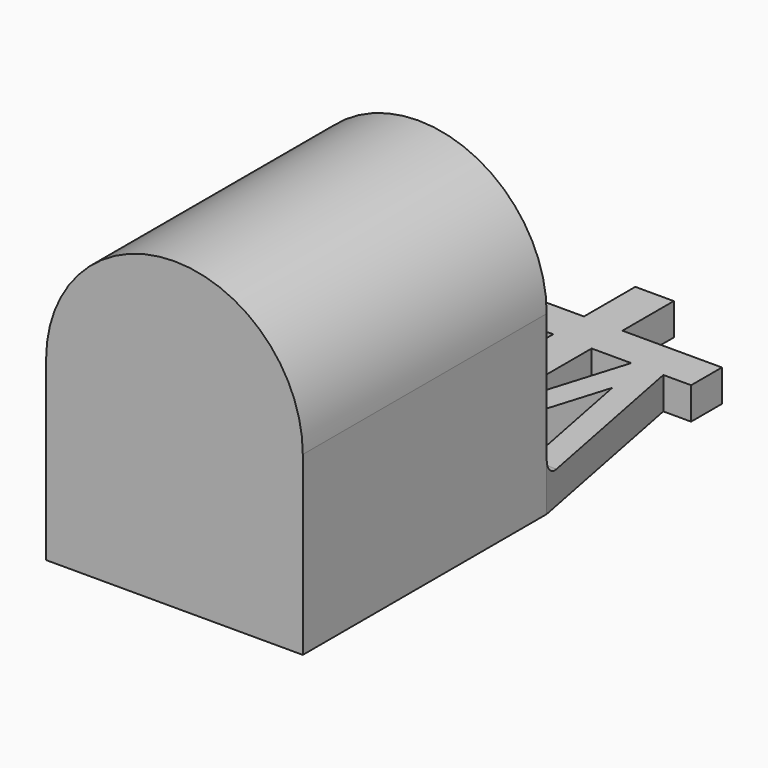
from build123d import *

# Parameters (mm, degrees)
F1_DEPTH  = 10
F3_DEPTH  = 100
F4_R      = 35
F5_DEPTH  = 90
F6_DEPTH  = 95.001
F7_R      = 5
F10_R     = 4
F11_DEPTH = 18


with BuildPart() as f1:
    # F0 (on Top) → F1 (new body)
    with BuildSketch(Plane.XY):
        Polygon((-6, 61.6815258077), (-6, 41.6815258077), (-37, 41.6815258077), (-37, 29.6815258077), (-28.3371814517, 29.6815258077), (-40, -30.3184741923), (-40, -125.3184741923), (0, -125.3184741923), (40, -125.3184741923), (40, -30.3184741923), (28.3371814517, 29.6815258077), (37, 29.6815258077), (37, 41.6815258077), (6, 41.6815258077), (6, 61.6815258077), (0, 61.6815258077), align=None)
        Polygon((-8.5239209836, -30.3184741923), (-32, -30.3184741923), (-22.8734250069, 16.6336838404), align=None, mode=Mode.SUBTRACT)
        Polygon((-18.3371814517, 29.6815258077), (-6, 29.6815258077), (-6, -10.686231312), align=None, mode=Mode.SUBTRACT)
        Polygon((6, -10.686231312), (6, 29.6815258077), (18.3371814517, 29.6815258077), align=None, mode=Mode.SUBTRACT)
        Polygon((22.8734250069, 16.6336838404), (32, -30.3184741923), (8.5239209836, -30.3184741923), align=None, mode=Mode.SUBTRACT)
    extrude(amount=F1_DEPTH)

    # F2 (on face) → F3 (join)
    with BuildSketch(Plane.XY.offset(10)):
        Polygon((-8.5239209836, -30.3184741923), (-40, -30.3184741923), (-40, -125.3184741923), (40, -125.3184741923), (40, -30.3184741923), (8.5239209836, -30.3184741923), align=None)
    extrude(amount=F3_DEPTH)

    # F4 (on face) → F5 (cut)
    with BuildSketch(Plane(origin=(0, -30.3184741923, 0), x_dir=(-1, 0, 0), z_dir=(0, 1, 0))):
        with Locations((0, 55)):
            Circle(F4_R)
    extrude(amount=-F5_DEPTH, mode=Mode.SUBTRACT)

    # F4 (on face) → F6 (cut, through all)
    with BuildSketch(Plane(origin=(0, -30.3184741923, 0), x_dir=(-1, 0, 0), z_dir=(0, 1, 0))):
        with BuildLine():
            ThreePointArc((-40, 55), (0, 95), (40, 55))
            Line((40, 55), (40, 110))
            Line((40, 110), (-40, 110))
            Line((-40, 110), (-40, 55))
        make_face()
    extrude(amount=-F6_DEPTH, mode=Mode.SUBTRACT)

    # F7
    f7_edges = [f1.edges().sort_by_distance(p)[0] for p in [
        (0, -30.318474, 10),
        (-8.523921, -30.318474, 5),
        (8.523921, -30.318474, 5),
        (36, -30.318474, 10),
        (32, -30.318474, 5),
        (-36, -30.318474, 10),
        (-32, -30.318474, 5),
    ]]
    fillet(f7_edges, radius=F7_R)

    # F10 (on face) → F11 (cut)
    with BuildSketch(Plane(origin=(0, 7.9203814519, 13.7185030901), x_dir=(1, 0, 0), z_dir=(0, 0.5, 0.8660254038))):
        with Locations((0, 44.4177682936)):
            Circle(F10_R)
    extrude(amount=F11_DEPTH, mode=Mode.SUBTRACT)


solid = f1.part
